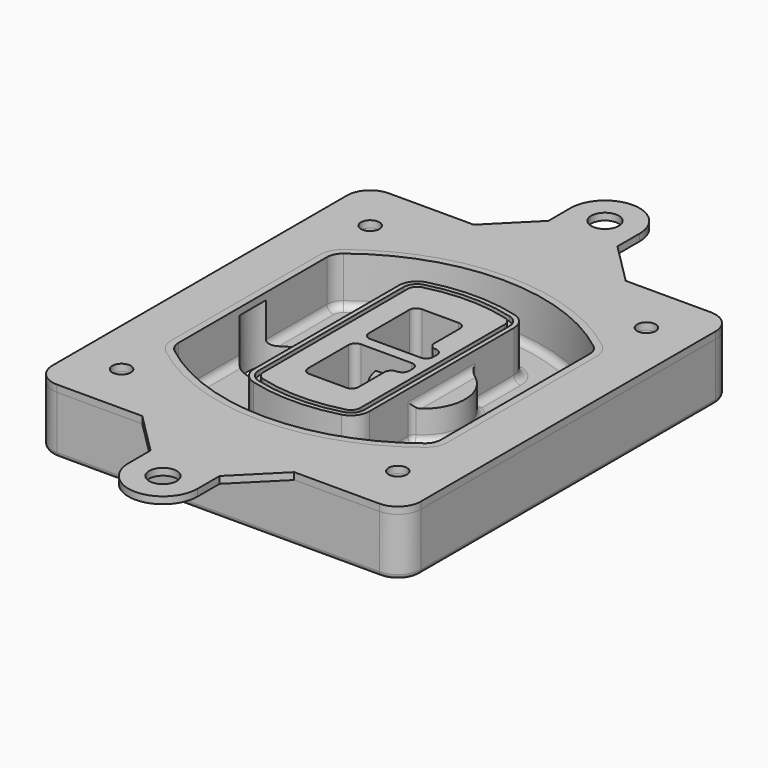
from build123d import *

# Parameters (mm, degrees)
F0_R      = 4
F1_DEPTH  = 25
F2_DEPTH  = 3
F3_DEPTH  = 18
F5_DEPTH  = 21
F6_DEPTH  = 2
F8_DEPTH  = 20
F9_DEPTH  = 16
F10_DEPTH = 25
F7_R      = 6
F7_R_2    = 4
F11_DEPTH = 6
F13_DEPTH = 9
F14_R     = 3
F15_R     = 2
F16_R     = 6
F16_R_2   = 4
F17_DEPTH = 3


# Not quite as in the source:
# - a feature names something its author has since deleted; it is built from what else it names


with BuildPart() as f1:
    # F0 (on Top) → F1 (new body)
    with BuildSketch(Plane.XY):
        with BuildLine():
            ThreePointArc((-80, -80), (-77.0710678119, -87.0710678119), (-70, -90))
            Line((-70, -90), (70, -90))
            ThreePointArc((70, -90), (77.0710678119, -87.0710678119), (80, -80))
            Line((80, -80), (80, 80))
            ThreePointArc((80, 80), (77.0710678119, 87.0710678119), (70, 90))
            Line((70, 90), (-70, 90))
            ThreePointArc((-70, 90), (-77.0710678119, 87.0710678119), (-80, 80))
            Line((-80, 80), (-80, -80))
        make_face()
        with Locations((-60, -67.5)):
            Circle(F0_R, mode=Mode.SUBTRACT)
        with Locations((60, -67.5)):
            Circle(F0_R, mode=Mode.SUBTRACT)
        with Locations((-60, 67.5)):
            Circle(F0_R, mode=Mode.SUBTRACT)
        with BuildLine():
            ThreePointArc((-64, 40.2934422872), (-62.5820384798, 46.4328484224), (-58.6153846154, 51.3286200352))
            ThreePointArc((-58.6153846154, 51.3286200352), (0, 71.5), (58.6153846154, 51.3286200352))
            ThreePointArc((58.6153846154, 51.3286200352), (62.5820384798, 46.4328484224), (64, 40.2934422872))
            Line((64, 40.2934422872), (64, -40.2934422872))
            ThreePointArc((64, -40.2934422872), (62.5820384798, -46.4328484224), (58.6153846154, -51.3286200352))
            ThreePointArc((58.6153846154, -51.3286200352), (0, -71.5), (-58.6153846154, -51.3286200352))
            ThreePointArc((-58.6153846154, -51.3286200352), (-62.5820384798, -46.4328484224), (-64, -40.2934422872))
            Line((-64, -40.2934422872), (-64, 40.2934422872))
        make_face(mode=Mode.SUBTRACT)
        with Locations((60, 67.5)):
            Circle(F0_R, mode=Mode.SUBTRACT)
        with BuildLine():
            ThreePointArc((58.6153846154, 51.3286200352), (0, 71.5), (-58.6153846154, 51.3286200352))
            ThreePointArc((-58.6153846154, 51.3286200352), (-62.5820384798, 46.4328484224), (-64, 40.2934422872))
            Line((-64, 40.2934422872), (-64, -40.2934422872))
            ThreePointArc((-64, -40.2934422872), (-62.5820384798, -46.4328484224), (-58.6153846154, -51.3286200352))
            ThreePointArc((-58.6153846154, -51.3286200352), (0, -71.5), (58.6153846154, -51.3286200352))
            ThreePointArc((58.6153846154, -51.3286200352), (62.5820384798, -46.4328484224), (64, -40.2934422872))
            Line((64, -40.2934422872), (64, 40.2934422872))
            ThreePointArc((64, 40.2934422872), (62.5820384798, 46.4328484224), (58.6153846154, 51.3286200352))
        make_face()
        with BuildLine():
            Line((-60, -40.2934422872), (-60, 40.2934422872))
            ThreePointArc((-60, 40.2934422872), (-58.9871703427, 44.6787323838), (-56.1538461538, 48.1757121072))
            ThreePointArc((-56.1538461538, 48.1757121072), (0, 67.5), (56.1538461538, 48.1757121072))
            ThreePointArc((56.1538461538, 48.1757121072), (58.9871703427, 44.6787323838), (60, 40.2934422872))
            Line((60, 40.2934422872), (60, -40.2934422872))
            ThreePointArc((60, -40.2934422872), (58.9871703427, -44.6787323838), (56.1538461538, -48.1757121072))
            ThreePointArc((56.1538461538, -48.1757121072), (0, -67.5), (-56.1538461538, -48.1757121072))
            ThreePointArc((-56.1538461538, -48.1757121072), (-58.9871703427, -44.6787323838), (-60, -40.2934422872))
        make_face(mode=Mode.SUBTRACT)
        with BuildLine():
            ThreePointArc((-56.1538461538, 48.1757121072), (-58.9871703427, 44.6787323838), (-60, 40.2934422872))
            Line((-60, 40.2934422872), (-60, -40.2934422872))
            ThreePointArc((-60, -40.2934422872), (-58.9871703427, -44.6787323838), (-56.1538461538, -48.1757121072))
            ThreePointArc((-56.1538461538, -48.1757121072), (0, -67.5), (56.1538461538, -48.1757121072))
            ThreePointArc((56.1538461538, -48.1757121072), (58.9871703427, -44.6787323838), (60, -40.2934422872))
            Line((60, -40.2934422872), (60, 40.2934422872))
            ThreePointArc((60, 40.2934422872), (58.9871703427, 44.6787323838), (56.1538461538, 48.1757121072))
            ThreePointArc((56.1538461538, 48.1757121072), (0, 67.5), (-56.1538461538, 48.1757121072))
        make_face()
        with BuildLine():
            ThreePointArc((54.3076923077, 45.8110311612), (56.2910192399, 43.3631453548), (57, 40.2934422872))
            Line((57, 40.2934422872), (57, -40.2934422872))
            ThreePointArc((57, -40.2934422872), (56.2910192399, -43.3631453548), (54.3076923077, -45.8110311612))
            ThreePointArc((54.3076923077, -45.8110311612), (0, -64.5), (-54.3076923077, -45.8110311612))
            ThreePointArc((-54.3076923077, -45.8110311612), (-56.2910192399, -43.3631453548), (-57, -40.2934422872))
            Line((-57, -40.2934422872), (-57, 40.2934422872))
            ThreePointArc((-57, 40.2934422872), (-56.2910192399, 43.3631453548), (-54.3076923077, 45.8110311612))
            ThreePointArc((-54.3076923077, 45.8110311612), (0, 64.5), (54.3076923077, 45.8110311612))
        make_face(mode=Mode.SUBTRACT)
        with BuildLine():
            Line((57, -40.2934422872), (57, 40.2934422872))
            ThreePointArc((57, 40.2934422872), (56.2910192399, 43.3631453548), (54.3076923077, 45.8110311612))
            ThreePointArc((54.3076923077, 45.8110311612), (0, 64.5), (-54.3076923077, 45.8110311612))
            ThreePointArc((-54.3076923077, 45.8110311612), (-56.2910192399, 43.3631453548), (-57, 40.2934422872))
            Line((-57, 40.2934422872), (-57, -40.2934422872))
            ThreePointArc((-57, -40.2934422872), (-56.2910192399, -43.3631453548), (-54.3076923077, -45.8110311612))
            ThreePointArc((-54.3076923077, -45.8110311612), (0, -64.5), (54.3076923077, -45.8110311612))
            ThreePointArc((54.3076923077, -45.8110311612), (56.2910192399, -43.3631453548), (57, -40.2934422872))
        make_face()
    extrude(amount=-F1_DEPTH)

    # F0 (on Top) → F2 (join)
    with BuildSketch(Plane.XY):
        with BuildLine():
            ThreePointArc((-56.1538461538, 48.1757121072), (-58.9871703427, 44.6787323838), (-60, 40.2934422872))
            Line((-60, 40.2934422872), (-60, -40.2934422872))
            ThreePointArc((-60, -40.2934422872), (-58.9871703427, -44.6787323838), (-56.1538461538, -48.1757121072))
            ThreePointArc((-56.1538461538, -48.1757121072), (0, -67.5), (56.1538461538, -48.1757121072))
            ThreePointArc((56.1538461538, -48.1757121072), (58.9871703427, -44.6787323838), (60, -40.2934422872))
            Line((60, -40.2934422872), (60, 40.2934422872))
            ThreePointArc((60, 40.2934422872), (58.9871703427, 44.6787323838), (56.1538461538, 48.1757121072))
            ThreePointArc((56.1538461538, 48.1757121072), (0, 67.5), (-56.1538461538, 48.1757121072))
        make_face()
        with BuildLine():
            ThreePointArc((54.3076923077, 45.8110311612), (56.2910192399, 43.3631453548), (57, 40.2934422872))
            Line((57, 40.2934422872), (57, -40.2934422872))
            ThreePointArc((57, -40.2934422872), (56.2910192399, -43.3631453548), (54.3076923077, -45.8110311612))
            ThreePointArc((54.3076923077, -45.8110311612), (0, -64.5), (-54.3076923077, -45.8110311612))
            ThreePointArc((-54.3076923077, -45.8110311612), (-56.2910192399, -43.3631453548), (-57, -40.2934422872))
            Line((-57, -40.2934422872), (-57, 40.2934422872))
            ThreePointArc((-57, 40.2934422872), (-56.2910192399, 43.3631453548), (-54.3076923077, 45.8110311612))
            ThreePointArc((-54.3076923077, 45.8110311612), (0, 64.5), (54.3076923077, 45.8110311612))
        make_face(mode=Mode.SUBTRACT)
    extrude(amount=F2_DEPTH)

    # F0 (on Top) → F3 (cut)
    with BuildSketch(Plane.XY):
        with BuildLine():
            Line((57, -40.2934422872), (57, 40.2934422872))
            ThreePointArc((57, 40.2934422872), (56.2910192399, 43.3631453548), (54.3076923077, 45.8110311612))
            ThreePointArc((54.3076923077, 45.8110311612), (0, 64.5), (-54.3076923077, 45.8110311612))
            ThreePointArc((-54.3076923077, 45.8110311612), (-56.2910192399, 43.3631453548), (-57, 40.2934422872))
            Line((-57, 40.2934422872), (-57, -40.2934422872))
            ThreePointArc((-57, -40.2934422872), (-56.2910192399, -43.3631453548), (-54.3076923077, -45.8110311612))
            ThreePointArc((-54.3076923077, -45.8110311612), (0, -64.5), (54.3076923077, -45.8110311612))
            ThreePointArc((54.3076923077, -45.8110311612), (56.2910192399, -43.3631453548), (57, -40.2934422872))
        make_face()
    extrude(amount=-F3_DEPTH, mode=Mode.SUBTRACT)

    # F4 (on face) → F5 (join, through all)
    with BuildSketch(Plane.XY.offset(3)):
        with BuildLine():
            ThreePointArc((-25, -39.2465276821), (-23.3511545998, -44.1109737193), (-19.0842911877, -46.9702398883))
            ThreePointArc((-19.0842911877, -46.9702398883), (0, -49.5), (19.0842911877, -46.9702398883))
            ThreePointArc((19.0842911877, -46.9702398883), (23.3511545998, -44.1109737193), (25, -39.2465276821))
            Line((25, -39.2465276821), (25, 39.2465276821))
            ThreePointArc((25, 39.2465276821), (23.3511545998, 44.1109737193), (19.0842911877, 46.9702398883))
            ThreePointArc((19.0842911877, 46.9702398883), (0, 49.5), (-19.0842911877, 46.9702398883))
            ThreePointArc((-19.0842911877, 46.9702398883), (-23.3511545998, 44.1109737193), (-25, 39.2465276821))
            Line((-25, 39.2465276821), (-25, -39.2465276821))
        make_face()
        with BuildLine():
            ThreePointArc((18.5632183908, 45.0393118368), (21.7633659499, 42.89486221), (23, 39.2465276821))
            Line((23, 39.2465276821), (23, -39.2465276821))
            ThreePointArc((23, -39.2465276821), (21.7633659499, -42.89486221), (18.5632183908, -45.0393118368))
            ThreePointArc((18.5632183908, -45.0393118368), (0, -47.5), (-18.5632183908, -45.0393118368))
            ThreePointArc((-18.5632183908, -45.0393118368), (-21.7633659499, -42.89486221), (-23, -39.2465276821))
            Line((-23, -39.2465276821), (-23, 39.2465276821))
            ThreePointArc((-23, 39.2465276821), (-21.7633659499, 42.89486221), (-18.5632183908, 45.0393118368))
            ThreePointArc((-18.5632183908, 45.0393118368), (0, 47.5), (18.5632183908, 45.0393118368))
        make_face(mode=Mode.SUBTRACT)
        with BuildLine():
            Line((23, -39.2465276821), (23, 39.2465276821))
            ThreePointArc((23, 39.2465276821), (21.7633659499, 42.89486221), (18.5632183908, 45.0393118368))
            ThreePointArc((18.5632183908, 45.0393118368), (0, 47.5), (-18.5632183908, 45.0393118368))
            ThreePointArc((-18.5632183908, 45.0393118368), (-21.7633659499, 42.89486221), (-23, 39.2465276821))
            Line((-23, 39.2465276821), (-23, -39.2465276821))
            ThreePointArc((-23, -39.2465276821), (-21.7633659499, -42.89486221), (-18.5632183908, -45.0393118368))
            ThreePointArc((-18.5632183908, -45.0393118368), (0, -47.5), (18.5632183908, -45.0393118368))
            ThreePointArc((18.5632183908, -45.0393118368), (21.7633659499, -42.89486221), (23, -39.2465276821))
        make_face()
        with BuildLine():
            ThreePointArc((18.0421455939, 43.1083837852), (20.1755772999, 41.6787507007), (21, 39.2465276821))
            Line((21, 39.2465276821), (21, -39.2465276821))
            ThreePointArc((21, -39.2465276821), (20.1755772999, -41.6787507007), (18.0421455939, -43.1083837852))
            ThreePointArc((18.0421455939, -43.1083837852), (0, -45.5), (-18.0421455939, -43.1083837852))
            ThreePointArc((-18.0421455939, -43.1083837852), (-20.1755772999, -41.6787507007), (-21, -39.2465276821))
            Line((-21, -39.2465276821), (-21, 39.2465276821))
            ThreePointArc((-21, 39.2465276821), (-20.1755772999, 41.6787507007), (-18.0421455939, 43.1083837852))
            ThreePointArc((-18.0421455939, 43.1083837852), (0, 45.5), (18.0421455939, 43.1083837852))
        make_face(mode=Mode.SUBTRACT)
        with BuildLine():
            Line((21, -39.2465276821), (21, 39.2465276821))
            ThreePointArc((21, 39.2465276821), (20.1755772999, 41.6787507007), (18.0421455939, 43.1083837852))
            ThreePointArc((18.0421455939, 43.1083837852), (0, 45.5), (-18.0421455939, 43.1083837852))
            ThreePointArc((-18.0421455939, 43.1083837852), (-20.1755772999, 41.6787507007), (-21, 39.2465276821))
            Line((-21, 39.2465276821), (-21, -39.2465276821))
            ThreePointArc((-21, -39.2465276821), (-20.1755772999, -41.6787507007), (-18.0421455939, -43.1083837852))
            ThreePointArc((-18.0421455939, -43.1083837852), (0, -45.5), (18.0421455939, -43.1083837852))
            ThreePointArc((18.0421455939, -43.1083837852), (20.1755772999, -41.6787507007), (21, -39.2465276821))
        make_face()
        with BuildLine():
            Line((-8, -2.5), (14, -2.5))
            ThreePointArc((14, -2.5), (16.1213203436, -3.3786796564), (17, -5.5))
            Line((17, -5.5), (17, -7.5))
            ThreePointArc((17, -7.5), (16.1213203436, -9.6213203436), (14, -10.5))
            ThreePointArc((14, -10.5), (11.8786796564, -11.3786796564), (11, -13.5))
            Line((11, -13.5), (11, -27.5))
            ThreePointArc((11, -27.5), (10.1213203436, -29.6213203436), (8, -30.5))
            Line((8, -30.5), (-8, -30.5))
            ThreePointArc((-8, -30.5), (-10.1213203436, -29.6213203436), (-11, -27.5))
            Line((-11, -27.5), (-11, -5.5))
            ThreePointArc((-11, -5.5), (-10.1213203436, -3.3786796564), (-8, -2.5))
        make_face(mode=Mode.SUBTRACT)
        with BuildLine():
            ThreePointArc((-8, 2.5), (-10.1213203436, 3.3786796564), (-11, 5.5))
            Line((-11, 5.5), (-11, 27.5))
            ThreePointArc((-11, 27.5), (-10.1213203436, 29.6213203436), (-8, 30.5))
            Line((-8, 30.5), (8, 30.5))
            ThreePointArc((8, 30.5), (10.1213203436, 29.6213203436), (11, 27.5))
            Line((11, 27.5), (11, 13.5))
            ThreePointArc((11, 13.5), (11.8786796564, 11.3786796564), (14, 10.5))
            ThreePointArc((14, 10.5), (16.1213203436, 9.6213203436), (17, 7.5))
            Line((17, 7.5), (17, 5.5))
            ThreePointArc((17, 5.5), (16.1213203436, 3.3786796564), (14, 2.5))
            Line((14, 2.5), (-8, 2.5))
        make_face(mode=Mode.SUBTRACT)
    extrude(amount=-F5_DEPTH)

    # F4 (on face) → F6 (cut)
    with BuildSketch(Plane.XY.offset(3)):
        with BuildLine():
            Line((23, -39.2465276821), (23, 39.2465276821))
            ThreePointArc((23, 39.2465276821), (21.7633659499, 42.89486221), (18.5632183908, 45.0393118368))
            ThreePointArc((18.5632183908, 45.0393118368), (0, 47.5), (-18.5632183908, 45.0393118368))
            ThreePointArc((-18.5632183908, 45.0393118368), (-21.7633659499, 42.89486221), (-23, 39.2465276821))
            Line((-23, 39.2465276821), (-23, -39.2465276821))
            ThreePointArc((-23, -39.2465276821), (-21.7633659499, -42.89486221), (-18.5632183908, -45.0393118368))
            ThreePointArc((-18.5632183908, -45.0393118368), (0, -47.5), (18.5632183908, -45.0393118368))
            ThreePointArc((18.5632183908, -45.0393118368), (21.7633659499, -42.89486221), (23, -39.2465276821))
        make_face()
        with BuildLine():
            ThreePointArc((18.0421455939, 43.1083837852), (20.1755772999, 41.6787507007), (21, 39.2465276821))
            Line((21, 39.2465276821), (21, -39.2465276821))
            ThreePointArc((21, -39.2465276821), (20.1755772999, -41.6787507007), (18.0421455939, -43.1083837852))
            ThreePointArc((18.0421455939, -43.1083837852), (0, -45.5), (-18.0421455939, -43.1083837852))
            ThreePointArc((-18.0421455939, -43.1083837852), (-20.1755772999, -41.6787507007), (-21, -39.2465276821))
            Line((-21, -39.2465276821), (-21, 39.2465276821))
            ThreePointArc((-21, 39.2465276821), (-20.1755772999, 41.6787507007), (-18.0421455939, 43.1083837852))
            ThreePointArc((-18.0421455939, 43.1083837852), (0, 45.5), (18.0421455939, 43.1083837852))
        make_face(mode=Mode.SUBTRACT)
    extrude(amount=-F6_DEPTH, mode=Mode.SUBTRACT)

    # F7 (on face) → F8 (join)
    with BuildSketch(Plane(origin=(0, 0, -25), x_dir=(1, 0, 0), z_dir=(0, 0, -1))):
        with BuildLine():
            ThreePointArc((3.28842436, 0), (16.7567035675, 13.4682792075), (30.224982775, 0))
            Line((30.224982775, 0), (35.224982775, 0))
            ThreePointArc((35.224982775, 0), (16.7567035675, 18.4682792075), (-1.71157564, 0))
            Line((-1.71157564, 0), (3.28842436, 0))
        make_face()
        with BuildLine():
            Line((3.28842436, 0), (30.224982775, 0))
            ThreePointArc((30.224982775, 0), (16.7567035675, 13.4682792075), (3.28842436, 0))
        make_face()
        with BuildLine():
            ThreePointArc((3.28842436, 0), (16.7567035675, -13.4682792075), (30.224982775, 0))
            Line((30.224982775, 0), (3.28842436, 0))
        make_face()
        with BuildLine():
            Line((35.224982775, 0), (30.224982775, 0))
            ThreePointArc((30.224982775, 0), (16.7567035675, -13.4682792075), (3.28842436, 0))
            Line((3.28842436, 0), (-1.71157564, 0))
            ThreePointArc((-1.71157564, 0), (16.7567035675, -18.4682792075), (35.224982775, 0))
        make_face()
    extrude(amount=-F8_DEPTH)

    # F7 (on face) → F9 (cut)
    with BuildSketch(Plane(origin=(0, 0, -25), x_dir=(1, 0, 0), z_dir=(0, 0, -1))):
        with BuildLine():
            Line((3.28842436, 0), (30.224982775, 0))
            ThreePointArc((30.224982775, 0), (16.7567035675, 13.4682792075), (3.28842436, 0))
        make_face()
        with BuildLine():
            ThreePointArc((3.28842436, 0), (16.7567035675, -13.4682792075), (30.224982775, 0))
            Line((30.224982775, 0), (3.28842436, 0))
        make_face()
    extrude(amount=-F9_DEPTH, mode=Mode.SUBTRACT)

    # F7 (on face) → F10 (cut)
    with BuildSketch(Plane(origin=(0, 0, -25), x_dir=(1, 0, 0), z_dir=(0, 0, -1))):
        with BuildLine():
            Line((-59.0318229325, 0), (-32.0952645175, 0))
            ThreePointArc((-32.0952645175, 0), (-45.563543725, 13.4682792075), (-59.0318229325, 0))
        make_face()
        with BuildLine():
            ThreePointArc((-59.0318229325, 0), (-45.563543725, -13.4682792075), (-32.0952645175, 0))
            Line((-32.0952645175, 0), (-59.0318229325, 0))
        make_face()
    extrude(amount=-F10_DEPTH, mode=Mode.SUBTRACT)

    # F7 (on face) → F11 (cut)
    with BuildSketch(Plane(origin=(0, 0, -25), x_dir=(1, 0, 0), z_dir=(0, 0, -1))):
        with Locations((60, -67.5)):
            Circle(F7_R)
        with Locations((60, -67.5)):
            Circle(F7_R_2, mode=Mode.SUBTRACT)
        with Locations((-60, -67.5)):
            Circle(F7_R)
        with Locations((-60, -67.5)):
            Circle(F7_R_2, mode=Mode.SUBTRACT)
        with Locations((-60, 67.5)):
            Circle(F7_R)
        with Locations((-60, 67.5)):
            Circle(F7_R_2, mode=Mode.SUBTRACT)
        with Locations((60, 67.5)):
            Circle(F7_R)
        with Locations((60, 67.5)):
            Circle(F7_R_2, mode=Mode.SUBTRACT)
    extrude(amount=-F11_DEPTH, mode=Mode.SUBTRACT)

    # F12 (on face) → F13 (cut, through all)
    with BuildSketch(Plane(origin=(0, 0, -9), x_dir=(1, 0, 0), z_dir=(0, 0, -1))):
        with BuildLine():
            Line((11, 13.5), (11, 17.5481537753))
            ThreePointArc((11, 17.5481537753), (2.5696536419, 11.8239143813), (-1.5415842455, 2.5))
            Line((-1.5415842455, 2.5), (3.5224848595, 2.5))
            ThreePointArc((3.5224848595, 2.5), (6.1857188154, 8.3455872281), (11.2536447004, 12.2927168648))
            ThreePointArc((11.2536447004, 12.2927168648), (11.0640958889, 12.8831798879), (11, 13.5))
        make_face()
        with BuildLine():
            ThreePointArc((11.2536447004, -12.2927168648), (6.1857188154, -8.3455872281), (3.5224848595, -2.5))
            Line((3.5224848595, -2.5), (-1.5415842455, -2.5))
            ThreePointArc((-1.5415842455, -2.5), (2.5696536419, -11.8239143813), (11, -17.5481537753))
            Line((11, -17.5481537753), (11, -13.5))
            ThreePointArc((11, -13.5), (11.0640958889, -12.8831798879), (11.2536447004, -12.2927168648))
        make_face()
        with BuildLine():
            ThreePointArc((11.2536447004, 12.2927168648), (6.1857188154, 8.3455872281), (3.5224848595, 2.5))
            Line((3.5224848595, 2.5), (14, 2.5))
            ThreePointArc((14, 2.5), (16.1213203436, 3.3786796564), (17, 5.5))
            Line((17, 5.5), (17, 7.5))
            ThreePointArc((17, 7.5), (16.1213203436, 9.6213203436), (14, 10.5))
            ThreePointArc((14, 10.5), (12.3601599782, 10.9878446101), (11.2536447004, 12.2927168648))
        make_face()
        with BuildLine():
            Line((14, -2.5), (3.5224848595, -2.5))
            ThreePointArc((3.5224848595, -2.5), (6.1857188154, -8.3455872281), (11.2536447004, -12.2927168648))
            ThreePointArc((11.2536447004, -12.2927168648), (12.3601599782, -10.9878446101), (14, -10.5))
            ThreePointArc((14, -10.5), (16.1213203436, -9.6213203436), (17, -7.5))
            Line((17, -7.5), (17, -5.5))
            ThreePointArc((17, -5.5), (16.1213203436, -3.3786796564), (14, -2.5))
        make_face()
    extrude(amount=F13_DEPTH, mode=Mode.SUBTRACT)

    # F14
    f14_edges = [f1.edges().sort_by_distance(p)[0] for p in [
        (-57, -23.703476, -18),
        (-57, 23.703476, -18),
        (25, 0, -5),
        (25, 16.526506, -11.5),
        (25, -16.526506, -11.5),
        (25, -27.886517, -18),
        (35.224983, 0, -18),
        (23.351155, -44.110974, -18),
        (0, -64.5, -18),
        (-56.291019, -43.363145, -18),
        (-56.291019, 43.363145, -18),
        (0, 64.5, -18),
        (56.291019, 43.363145, -18),
        (57, 0, -18),
        (56.291019, -43.363145, -18),
        (-23.351155, 44.110974, -18),
        (0, 49.5, -18),
        (-25, 0, -18),
        (23.351155, 44.110974, -18),
        (-23.351155, -44.110974, -18),
        (25, 27.886517, -18),
        (0, -49.5, -18),
    ]]
    fillet(f14_edges, radius=F14_R)

    # F15
    f15_edges = [f1.edges().sort_by_distance(p)[0] for p in [
        (0, -90, -25),
        (-77.071068, -87.071068, -25),
        (-80, 0, -25),
        (-77.071068, 87.071068, -25),
        (77.071068, -87.071068, -25),
        (0, 90, -25),
        (80, 0, -25),
        (77.071068, 87.071068, -25),
    ]]
    fillet(f15_edges, radius=F15_R)


with BuildPart() as f17:
    # F16 (on face) → F17 (new body, through all)
    with BuildSketch(Plane.XY):
        with BuildLine():
            Line((15, 108), (15, 120))
            ThreePointArc((15, 120), (0, 135), (-15, 120))
            Line((-15, 120), (-15, 108))
            Line((-15, 108), (-33, 90))
            Line((-33, 90), (33, 90))
            Line((33, 90), (15, 108))
        make_face()
        with Locations((0, 120)):
            Circle(F16_R, mode=Mode.SUBTRACT)
        with BuildLine():
            Line((70, 90), (33, 90))
            Line((33, 90), (-33, 90))
            Line((-33, 90), (-70, 90))
            ThreePointArc((-70, 90), (-77.0710678119, 87.0710678119), (-80, 80))
            Line((-80, 80), (-80, -80))
            ThreePointArc((-80, -80), (-77.0710678119, -87.0710678119), (-70, -90))
            Line((-70, -90), (-33, -90))
            Line((-33, -90), (33, -90))
            Line((33, -90), (70, -90))
            ThreePointArc((70, -90), (77.0710678119, -87.0710678119), (80, -80))
            Line((80, -80), (80, 80))
            ThreePointArc((80, 80), (77.0710678119, 87.0710678119), (70, 90))
        make_face()
        with Locations((-60, -67.5)):
            Circle(F16_R_2, mode=Mode.SUBTRACT)
        with Locations((60, -67.5)):
            Circle(F16_R_2, mode=Mode.SUBTRACT)
        with Locations((-60, 67.5)):
            Circle(F16_R_2, mode=Mode.SUBTRACT)
        with BuildLine():
            ThreePointArc((-60, 40.2934422872), (-58.9871703427, 44.6787323838), (-56.1538461538, 48.1757121072))
            ThreePointArc((-56.1538461538, 48.1757121072), (0, 67.5), (56.1538461538, 48.1757121072))
            ThreePointArc((56.1538461538, 48.1757121072), (58.9871703427, 44.6787323838), (60, 40.2934422872))
            Line((60, 40.2934422872), (60, -40.2934422872))
            ThreePointArc((60, -40.2934422872), (58.9871703427, -44.6787323838), (56.1538461538, -48.1757121072))
            ThreePointArc((56.1538461538, -48.1757121072), (0, -67.5), (-56.1538461538, -48.1757121072))
            ThreePointArc((-56.1538461538, -48.1757121072), (-58.9871703427, -44.6787323838), (-60, -40.2934422872))
            Line((-60, -40.2934422872), (-60, 40.2934422872))
        make_face(mode=Mode.SUBTRACT)
        with Locations((60, 67.5)):
            Circle(F16_R_2, mode=Mode.SUBTRACT)
        with BuildLine():
            Line((15, -108), (33, -90))
            Line((33, -90), (-33, -90))
            Line((-33, -90), (-15, -108))
            Line((-15, -108), (-15, -120))
            ThreePointArc((-15, -120), (0, -135), (15, -120))
            Line((15, -120), (15, -108))
        make_face()
        with Locations((0, -120)):
            Circle(F16_R, mode=Mode.SUBTRACT)
    extrude(amount=F17_DEPTH)


solid = Compound([f1.part, f17.part])
